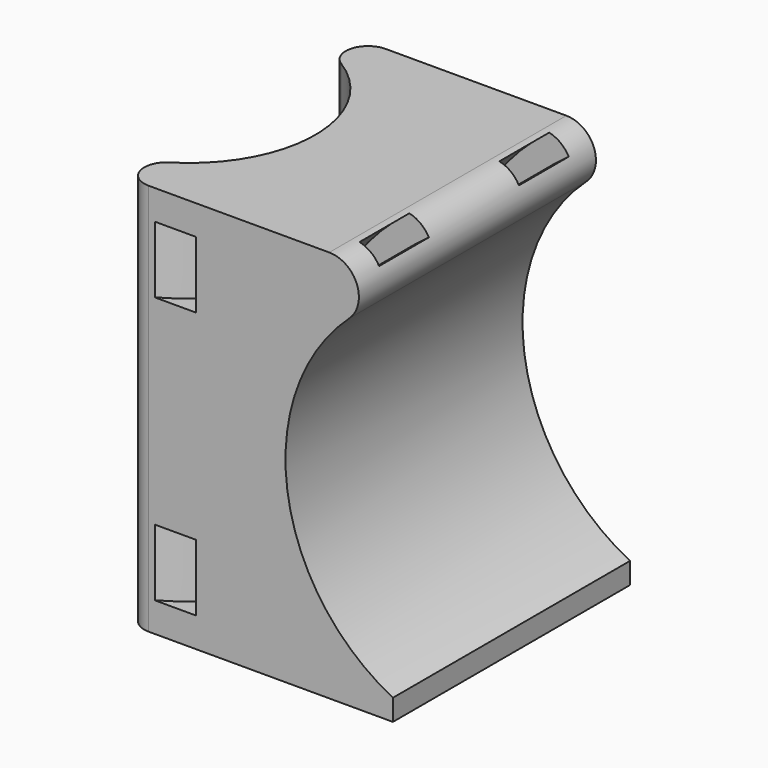
from build123d import *

# Parameters (mm, degrees)
F1_DEPTH      = 12.7
F4_DEPTH      = 16.8285
F4_DEPTH_BACK = 16.8285
F5_R          = 2.54
F6_W          = 5.334
F6_H          = 2.032
F8_W          = 7.62
F8_H          = 2.54
F9_DEPTH      = 12.701
F9_DEPTH_BACK = 12.701
F10_W         = 2.032
F10_H         = 5.715
F13_DEPTH     = 33.656
F14_R         = 1.90499


# Not quite as in the source:
# - a fillet or chamfer is up to 0.001 mm smaller than in the source, because OpenCascade refuses the exact size


with BuildPart() as f1:
    # F0 (on Front) → F1 (new body, symmetric)
    with BuildSketch(Plane.XZ):
        with BuildLine():
            Line((0, 16.8275), (0, -16.8275))
            Line((0, -16.8275), (35.2425, -16.8275))
            ThreePointArc((35.2425, -16.8275), (18.415, 0), (35.2425, 16.8275))
            Line((35.2425, 16.8275), (0, 16.8275))
        make_face()
    extrude(amount=F1_DEPTH, both=True)

    # F3 (on Top) → F4 (cut, two sides)
    with BuildSketch(Plane.XY) as f4_sk:
        with BuildLine():
            Line((0, 10.795), (0, -10.795))
            ThreePointArc((0, -10.795), (10.795, 0), (0, 10.795))
        make_face()
    extrude(amount=-F4_DEPTH, mode=Mode.SUBTRACT)
    extrude(f4_sk.sketch, amount=F4_DEPTH_BACK, mode=Mode.SUBTRACT)

    # F5
    f5_edges = [f1.edges().sort_by_distance(p)[0] for p in [
        (35.2425, 0, 16.8275),
    ]]
    fillet(f5_edges, radius=F5_R)

    # F6 (on offset) → F7 (revolve, cut)
    with BuildSketch(Plane.YZ.offset(32.7025)):
        with Locations((7.493, 19.7485)):
            Rectangle(F6_W, F6_H)
        with Locations((-7.493, 19.7485)):
            Rectangle(F6_W, F6_H)
    revolve(axis=Axis((35.2425, 0, 0), (0, -1, 0)), mode=Mode.SUBTRACT)

    # F8 (on Front) → F9 (cut, two sides)
    with BuildSketch(Plane.XZ) as f9_sk:
        with Locations((31.4325, -15.5575)):
            Rectangle(F8_W, F8_H)
    extrude(amount=F9_DEPTH, mode=Mode.SUBTRACT)
    extrude(f9_sk.sketch, amount=-F9_DEPTH_BACK, mode=Mode.SUBTRACT)

    # F10 (on Right) → F11 (revolve, cut)
    with BuildSketch(Plane.YZ):
        with Locations((-15.621, 11.43)):
            Rectangle(F10_W, F10_H)
        with Locations((-15.621, -11.43)):
            Rectangle(F10_W, F10_H)
    revolve(axis=Axis((0, 0, 0), (0, 0, 1)), mode=Mode.SUBTRACT)

    # F12 (on face) → F13 (cut, through all)
    with BuildSketch(Plane.XY.offset(16.8275)):
        Polygon((5.6866191131, 9.17575), (0, 12.7), (0, 9.17575), align=None)
        Polygon((5.6866191131, -9.17575), (0, -9.17575), (0, -12.7), align=None)
    extrude(amount=-F13_DEPTH, mode=Mode.SUBTRACT)

    # F14 (radius 1.905 in the source; OpenCascade refuses exactly that, so slightly less here)
    f14_edges = [f1.edges().sort_by_distance(p)[0] for p in [
        (0, 12.7, 0),
        (0, -12.7, 0),
    ]]
    fillet(f14_edges, radius=F14_R)


solid = f1.part
